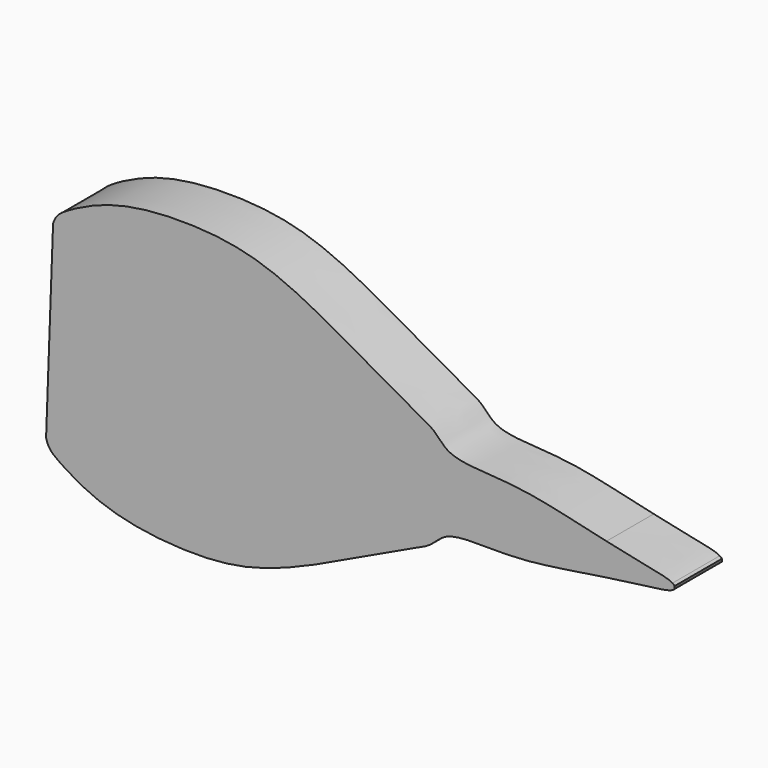
from build123d import *

# Parameters (mm, degrees)
F1_DEPTH = 10


with BuildPart() as f1:
    # F0 (on Front) → F1 (new body)
    with BuildSketch(Plane.XZ):
        with BuildLine():
            add(Edge.make_bspline(
                [(-43.2739737539, 19.3286379981), (-42.8717910323, 20.6443938488), (-41.2670866914, 21.9607246818), (-33.1050259673, 26.1698144492), (-20.4782941502, 27.1660016518), (-7.9180102102, 25.6432503479), (5.0492344453, 18.8178845805), (16.8426971438, 11.7818486723), (21.5410823221, 9.5845389909), (23.7573944562, 6.0271395456), (33.9663222046, 6.0122157554), (41.6732644409, 4.4779816736), (47.9916737559, 2.9982979686), (50.4361293155, 2.4450533648)],
                knots=[0.2096114324, 0.2096114324, 0.2096114324, 0.2096114324, 0.2372253632, 0.282305002, 0.3374939232, 0.3919156422, 0.4515775986, 0.5086523402, 0.5423950946, 0.5712274702, 0.6183035523, 0.6670425092, 0.6989923434, 0.6989923434, 0.6989923434, 0.6989923434], degree=3))
            Line((-43.2739737539, 19.3286379981), (-43.8562949661, 3.456262298))
            Line((-43.8562949661, 3.456262298), (-43.866463093, 3.1791088515))
            Line((-43.866463093, 3.1791088515), (61.9723973752, -0.7038772044))
            Line((61.9723973752, -0.7038772044), (61.9779187996, -0.5533792985))
            add(Edge.make_bspline(
                [(61.9779187996, -0.5533792985), (61.9043423038, -0.4347153333), (61.7777869789, -0.2956526047), (61.614568699, -0.1598779548)],
                knots=[0.7844933866, 0.7844933866, 0.7844933866, 0.7844933866, 0.7922828741, 0.7922828741, 0.7922828741, 0.7922828741], degree=3))
            add(Edge.make_bspline(
                [(50.4361293155, 2.4450533648), (52.1557640437, 2.0558547843), (56.6990812586, 1.0537255108), (60.587418179, 0.4072656539), (61.5305184171, -0.106596957), (61.614568699, -0.1598779548)],
                knots=[0.6989923434, 0.6989923434, 0.6989923434, 0.6989923434, 0.7214685321, 0.7593724987, 0.7638050529, 0.7638050529, 0.7638050529, 0.7638050529], degree=3))
        make_face()
        with BuildLine():
            Line((-43.866463093, 3.1791088515), (-43.8766312199, 2.9019554051))
            Line((-43.8766312199, 2.9019554051), (-44.4589524321, -12.9704202951))
            add(Edge.make_bspline(
                [(-44.4589524321, -12.9704202951), (-44.1542653031, -14.3121095861), (-42.650331497, -15.7424892526), (-34.8186419571, -20.5383531877), (-22.2988527346, -22.4571088129), (-9.6607529946, -21.8588286533), (3.7717720363, -16.0020101391), (16.0491078911, -9.8490768524), (20.8958739527, -8.001956969), (23.366902701, -4.6165253548), (33.5494787592, -5.3497192653), (41.3481257392, -4.3843498373), (47.757975395, -3.3716368828), (50.2363993771, -2.9990014855)],
                knots=[0.2096114324, 0.2096114324, 0.2096114324, 0.2096114324, 0.2372253632, 0.282305002, 0.3374939232, 0.3919156422, 0.4515775986, 0.5086523402, 0.5423950946, 0.5712274702, 0.6183035523, 0.6670425092, 0.6989923434, 0.6989923434, 0.6989923434, 0.6989923434], degree=3))
            add(Edge.make_bspline(
                [(50.2363993771, -2.9990014855), (51.9799303381, -2.7368585443), (56.5844663162, -2.0703431109), (60.5097205041, -1.7105460656), (61.4879395595, -1.2671722713), (61.5756681453, -1.2201934479)],
                knots=[0.6989923434, 0.6989923434, 0.6989923434, 0.6989923434, 0.7214685321, 0.7593724987, 0.7638050529, 0.7638050529, 0.7638050529, 0.7638050529], degree=3))
            add(Edge.make_bspline(
                [(61.9668759507, -0.8543751103), (61.884801939, -0.9673286138), (61.7483967681, -1.0967439225), (61.5756681453, -1.2201934479)],
                knots=[0.7844933866, 0.7844933866, 0.7844933866, 0.7844933866, 0.7922828741, 0.7922828741, 0.7922828741, 0.7922828741], degree=3))
            Line((61.9668759507, -0.8543751103), (61.9723973752, -0.7038772044))
            Line((61.9723973752, -0.7038772044), (-43.866463093, 3.1791088515))
        make_face()
        with BuildLine():
            add(Edge.make_bspline(
                [(61.614568699, -0.1598779548), (61.7949898213, -0.2742501756), (61.9077194324, -0.3862288488), (61.9805835524, -0.4807459177)],
                knots=[0.7638050529, 0.7638050529, 0.7638050529, 0.7638050529, 0.7733199098, 0.7733199098, 0.7733199098, 0.7733199098], degree=3))
            add(Edge.make_bspline(
                [(61.9779187996, -0.5533792985), (61.9043423038, -0.4347153333), (61.7777869789, -0.2956526047), (61.614568699, -0.1598779548)],
                knots=[0.7844933866, 0.7844933866, 0.7844933866, 0.7844933866, 0.7922828741, 0.7922828741, 0.7922828741, 0.7922828741], degree=3))
            Line((61.9779187996, -0.5533792985), (61.9805835524, -0.4807459177))
        make_face()
        with BuildLine():
            Line((61.9642111979, -0.9270084911), (61.9668759507, -0.8543751103))
            add(Edge.make_bspline(
                [(61.9668759507, -0.8543751103), (61.884801939, -0.9673286138), (61.7483967681, -1.0967439225), (61.5756681453, -1.2201934479)],
                knots=[0.7844933866, 0.7844933866, 0.7844933866, 0.7844933866, 0.7922828741, 0.7922828741, 0.7922828741, 0.7922828741], degree=3))
            add(Edge.make_bspline(
                [(61.5756681453, -1.2201934479), (61.7639850615, -1.1193493835), (61.8846170541, -1.0159322145), (61.9642111979, -0.9270084911)],
                knots=[0.7638050529, 0.7638050529, 0.7638050529, 0.7638050529, 0.7733199098, 0.7733199098, 0.7733199098, 0.7733199098], degree=3))
        make_face()
    extrude(amount=F1_DEPTH)


solid = f1.part
